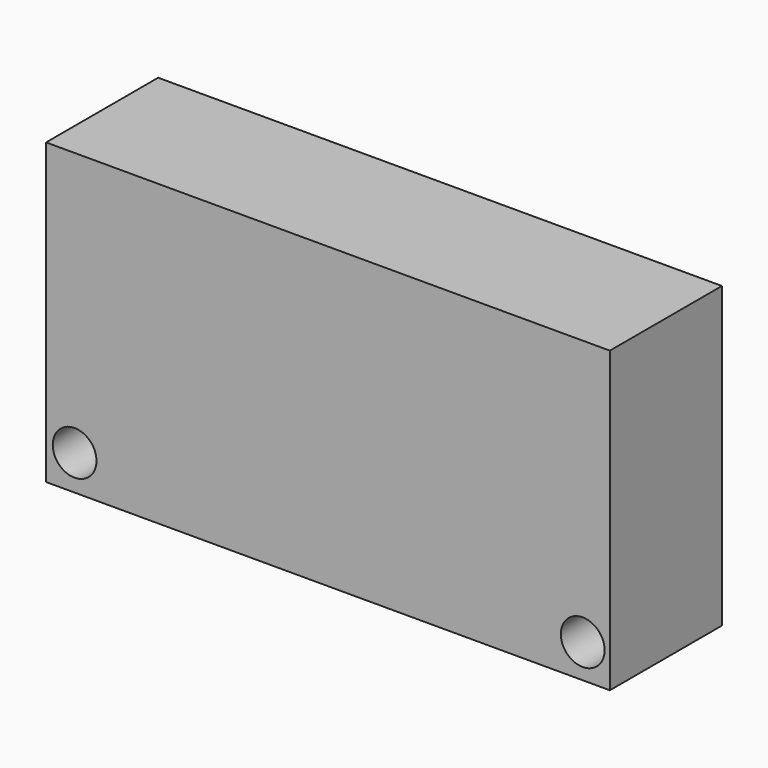
from build123d import *

# Parameters (mm, degrees)
F0_W     = 81.7696005106
F0_H     = 43.3689393103
F1_DEPTH = 25.4
F3_D     = 6.35
F3_DEPTH = 12.7
F3_TIP   = 1.9077324654
F5_SIZE  = 5.08


# Not quite as in the source:
# - the program builds the solid bodies; features that only make, move or delete a surface that nothing else refers to are left out


with BuildPart() as f1:
    # F0 (on Front) → F1 (new body)
    with BuildSketch(Plane.XZ):
        with Locations((-0.1035071909, 21.6844696552)):
            Rectangle(F0_W, F0_H)
    extrude(amount=-F1_DEPTH)

    # F3
    with Locations(Plane.XZ):
        with Locations((36.8480719626, 4.8647737131), (-36.8480719626, 5.071785301)):
            Hole(F3_D / 2, depth=F3_DEPTH)
            with Locations((0, 0, -(F3_DEPTH + F3_TIP / 2))):  # 118° drill point
                Cone(0, F3_D / 2, F3_TIP, mode=Mode.SUBTRACT)

    # F5
    f5_edges = [f1.edges().sort_by_distance(p)[0] for p in [
        (-40.988307, 25.4, 21.68447),
        (-0.103507, 25.4, 0),
        (40.781293, 25.4, 21.68447),
        (-0.103507, 25.4, 43.368939),
    ]]
    chamfer(f5_edges, length=F5_SIZE)


solid = f1.part
